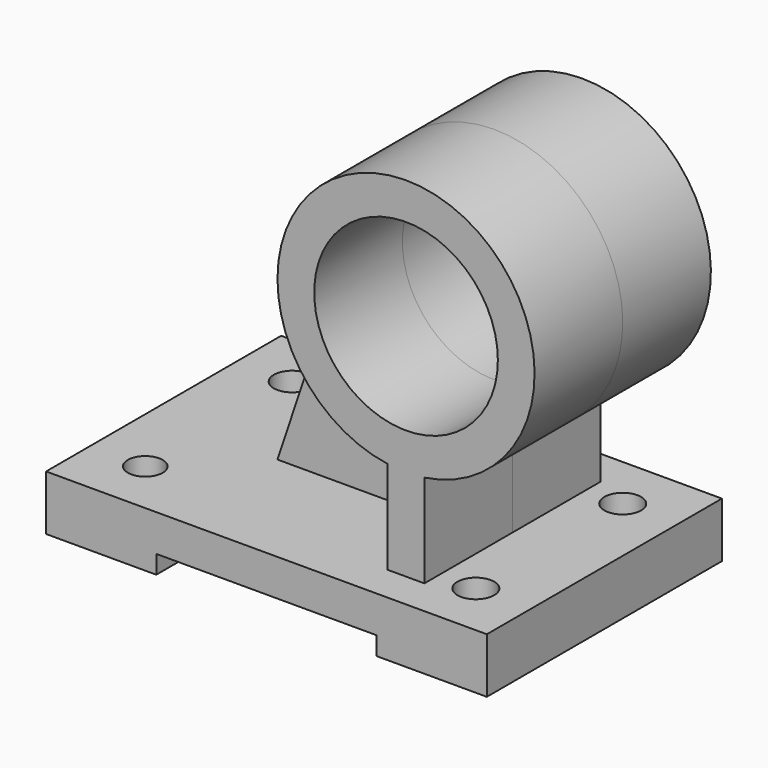
from build123d import *

# Parameters (mm, degrees)
F1_DEPTH      = 40
F1_DEPTH_BACK = 40
F2_DEPTH      = 5
F2_DEPTH_BACK = 5
F0_R          = 25
F3_DEPTH      = 30
F3_DEPTH_BACK = 30
F4_R          = 5
F4_R_2        = 4.7490283211
F5_DEPTH      = 25
F6_R          = 5
F7_DEPTH      = 25


with BuildPart() as f1:
    # F0 (on Front) → F1 (new body, two sides)
    with BuildSketch(Plane.XZ) as f1_sk:
        Polygon((60, -7.5), (60, 7.5), (35, 7.5), (25, 7.5), (-25, 7.5), (-60, 7.5), (-60, -7.5), (-30, -7.5), (-30, -2.5), (30, -2.5), (30, -7.5), align=None)
    extrude(amount=F1_DEPTH)
    extrude(f1_sk.sketch, amount=-F1_DEPTH_BACK)

    # F4 (on face) → F5 (cut)
    with BuildSketch(Plane.XY.offset(7.5)):
        with Locations((-45, 25)):
            Circle(F4_R)
        with Locations((-45, -25)):
            Circle(F4_R_2)
    extrude(amount=-F5_DEPTH, mode=Mode.SUBTRACT)

    # F6 (on face) → F7 (cut)
    with BuildSketch(Plane.XY.offset(7.5)):
        with Locations((45, -25)):
            Circle(F6_R)
        with Locations((45, 25)):
            Circle(F6_R)
    extrude(amount=-F7_DEPTH, mode=Mode.SUBTRACT)


with BuildPart() as f2:
    # F0 (on Front) → F2 (new body, two sides)
    with BuildSketch(Plane.XZ) as f2_sk:
        with BuildLine():
            Line((-25, 7.5), (25, 7.5))
            Line((25, 7.5), (25, 32.8589838486))
            ThreePointArc((25, 32.8589838486), (3.55471315, 44.573011462), (-4.9999800814, 67.462659662))
            Line((-4.9999800814, 67.462659662), (-25, 7.5))
        make_face()
    extrude(amount=F2_DEPTH)
    extrude(f2_sk.sketch, amount=-F2_DEPTH_BACK)

    # F0 (on Front) → F3 (join, two sides)
    with BuildSketch(Plane.XZ) as f3_sk:
        with BuildLine():
            ThreePointArc((25, 32.8589838486), (30, 32.5), (35, 32.8589838486))
            ThreePointArc((35, 32.8589838486), (56.4575131106, 44.5871215252), (65, 67.5))
            ThreePointArc((65, 67.5), (29.9813298283, 102.4999950204), (-4.9999800814, 67.462659662))
            ThreePointArc((-4.9999800814, 67.462659662), (3.55471315, 44.573011462), (25, 32.8589838486))
        make_face()
        with Locations((30, 67.5)):
            Circle(F0_R, mode=Mode.SUBTRACT)
        with BuildLine():
            Line((25, 7.5), (35, 7.5))
            Line((35, 7.5), (35, 32.8589838486))
            ThreePointArc((35, 32.8589838486), (30, 32.5), (25, 32.8589838486))
            Line((25, 32.8589838486), (25, 7.5))
        make_face()
    extrude(amount=F3_DEPTH)
    extrude(f3_sk.sketch, amount=-F3_DEPTH_BACK)


solid = Compound([f1.part, f2.part])
